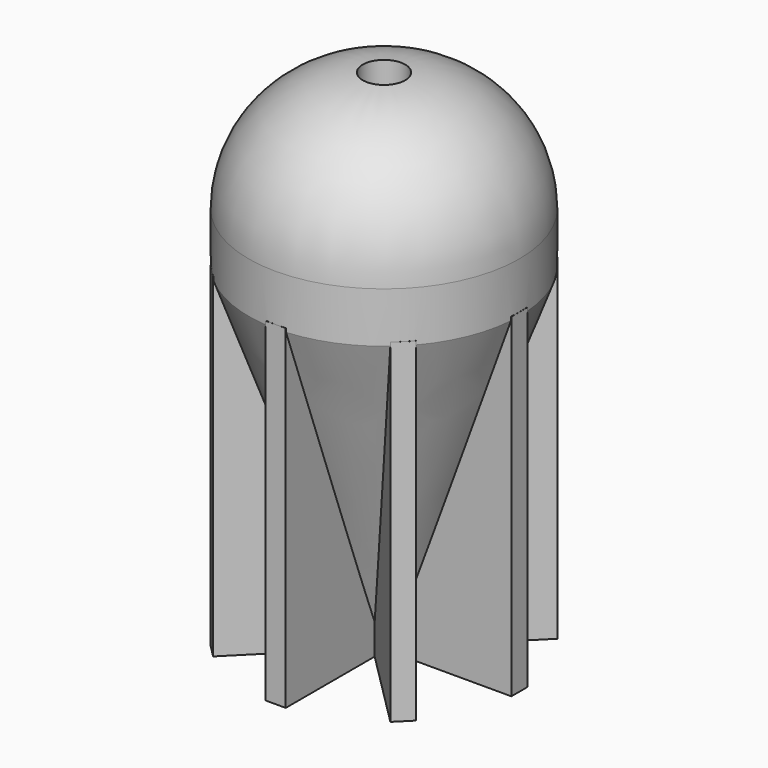
from build123d import *

# Parameters (mm, degrees)
F0_R      = 20.25
F1_DEPTH  = 75
F2_SIZE2  = 49.4545935502
F2_SIZE   = 18
F3_R      = 18
F7_E11_W  = 20.25
F7_E11_H  = 50
F14_DEPTH = 1.5
F9_E17_W  = 20.25
F9_E17_H  = 50
F15_DEPTH = 1.5
F9_E13_W  = 20.25
F9_E13_H  = 50
F16_DEPTH = 1.5
F11_E21_W = 20.25
F11_E21_H = 50
F17_DEPTH = 1.5
F11_E20_W = 20.25
F11_E20_H = 50
F18_DEPTH = 1.5
F13_E23_W = 20.25
F13_E23_H = 50
F19_DEPTH = 1.5
F5_E6_W   = 20.25
F5_E6_H   = 50
F20_DEPTH = 1.5
F13_E24_W = 20.25
F13_E24_H = 50
F21_DEPTH = 1.5
F22_R     = 3.175
F22_R_2   = 2.25
F23_DEPTH = 25


with BuildPart() as f1:
    # F0 (on Top) → F1 (new body)
    with BuildSketch(Plane.XY):
        Circle(F0_R)
    extrude(amount=F1_DEPTH)

    # F2
    f2_edges = [f1.edges().sort_by_distance(p)[0] for p in [
        (-20.25, 0, 0),
    ]]
    f2_side = f1.faces().sort_by_distance((0, 0, 0))[0]
    chamfer(f2_edges, length=F2_SIZE, length2=F2_SIZE2, reference=f2_side)

    # F3
    f3_edges = [f1.edges().sort_by_distance(p)[0] for p in [
        (-20.25, 0, 75),
    ]]
    fillet(f3_edges, radius=F3_R)

    # F7_E11 (on explicit) → F14 (join, symmetric)
    with BuildSketch(Plane.YZ):
        with Locations((10.125, 25)):
            Rectangle(F7_E11_W, F7_E11_H)
    extrude(amount=F14_DEPTH, both=True)

    # F9_E17 (on explicit) → F15 (join, symmetric)
    with BuildSketch(Plane(origin=(0, 0, 0), x_dir=(-0.7071067812, 0.7071067812, 0), z_dir=(0.7071067812, 0.7071067812, 0))):
        with Locations((10.125, 25)):
            Rectangle(F9_E17_W, F9_E17_H)
    extrude(amount=F15_DEPTH, both=True)

    # F9_E13 (on explicit) → F16 (join, symmetric)
    with BuildSketch(Plane(origin=(0, 0, 0), x_dir=(-1, 0, 0), z_dir=(0, 1, 0))):
        with Locations((10.125, 25)):
            Rectangle(F9_E13_W, F9_E13_H)
    extrude(amount=F16_DEPTH, both=True)

    # F11_E21 (on explicit) → F17 (join, symmetric)
    with BuildSketch(Plane(origin=(0, 0, 0), x_dir=(-0.7071067812, -0.7071067812, 0), z_dir=(-0.7071067812, 0.7071067812, 0))):
        with Locations((10.125, 25)):
            Rectangle(F11_E21_W, F11_E21_H)
    extrude(amount=F17_DEPTH, both=True)

    # F11_E20 (on explicit) → F18 (join, symmetric)
    with BuildSketch(Plane(origin=(0, 0, 0), x_dir=(0, -1, 0), z_dir=(-1, 0, 0))):
        with Locations((10.125, 25)):
            Rectangle(F11_E20_W, F11_E20_H)
    extrude(amount=F18_DEPTH, both=True)

    # F13_E23 (on explicit) → F19 (join, symmetric)
    with BuildSketch(Plane.XZ):
        with Locations((10.125, 25)):
            Rectangle(F13_E23_W, F13_E23_H)
    extrude(amount=F19_DEPTH, both=True)

    # F5_E6 (on explicit) → F20 (join, symmetric)
    with BuildSketch(Plane(origin=(0, 0, 0), x_dir=(0.7071067812, -0.7071067812, 0), z_dir=(-0.7071067812, -0.7071067812, 0))):
        with Locations((10.125, 25)):
            Rectangle(F5_E6_W, F5_E6_H)
    extrude(amount=F20_DEPTH, both=True)

    # F13_E24 (on explicit) → F21 (join, symmetric)
    with BuildSketch(Plane(origin=(0, 0, 0), x_dir=(0.7071067812, 0.7071067812, 0), z_dir=(0.7071067812, -0.7071067812, 0))):
        with Locations((10.125, 25)):
            Rectangle(F13_E24_W, F13_E24_H)
    extrude(amount=F21_DEPTH, both=True)

    # F22 (on face) → F23 (cut)
    with BuildSketch(Plane.XY.offset(75)):
        Circle(F22_R)
        Circle(F22_R_2, mode=Mode.SUBTRACT)
        Circle(F22_R_2)
    extrude(amount=-F23_DEPTH, mode=Mode.SUBTRACT)


solid = f1.part
